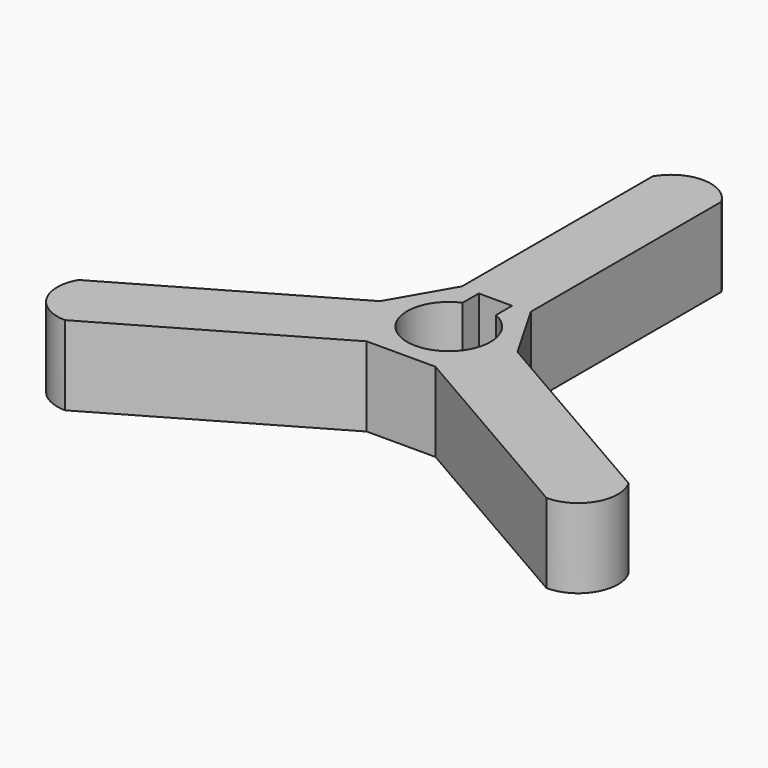
from build123d import *

# Parameters (mm, degrees)
F2_DEPTH = 9.525


# Not quite as in the source:
# - a variable given as a bare number and used for a length is read in inches; the dataset says mm whatever the document's units were


with BuildPart() as f2:
    # F1 (on Top) → F2 (new body)
    with BuildSketch(Plane.XY):
        with BuildLine():
            Line((4.1244459855, 7.14375), (4.1244459855, 35.71875))
            ThreePointArc((4.1244459855, 35.71875), (0, 38.1), (-4.1244459855, 35.71875))
            Line((-4.1244459855, 35.71875), (-4.1244459855, 7.14375))
            Line((-4.1244459855, 7.14375), (-8.248891971, 0))
            Line((-8.248891971, 0), (-32.9955678842, -14.2875))
            ThreePointArc((-32.9955678842, -14.2875), (-32.9955678842, -19.05), (-28.8711218987, -21.43125))
            Line((-28.8711218987, -21.43125), (-4.1244459855, -7.14375))
            Line((-4.1244459855, -7.14375), (4.1244459855, -7.14375))
            Line((4.1244459855, -7.14375), (28.8711218987, -21.43125))
            ThreePointArc((28.8711218987, -21.43125), (32.9955678842, -19.05), (32.9955678842, -14.2875))
            Line((32.9955678842, -14.2875), (8.248891971, 0))
            Line((8.248891971, 0), (4.1244459855, 7.14375))
        make_face()
        with BuildLine():
            ThreePointArc((2, 4.582575695), (4.1833001327, 2.7386127875), (5, 0))
            ThreePointArc((5, 0), (-2.7386127875, -4.1833001327), (-2, 4.582575695))
            Line((-2, 4.582575695), (-2, 7))
            Line((-2, 7), (2, 7))
            Line((2, 7), (2, 4.582575695))
        make_face(mode=Mode.SUBTRACT)
    extrude(amount=F2_DEPTH)


solid = f2.part
